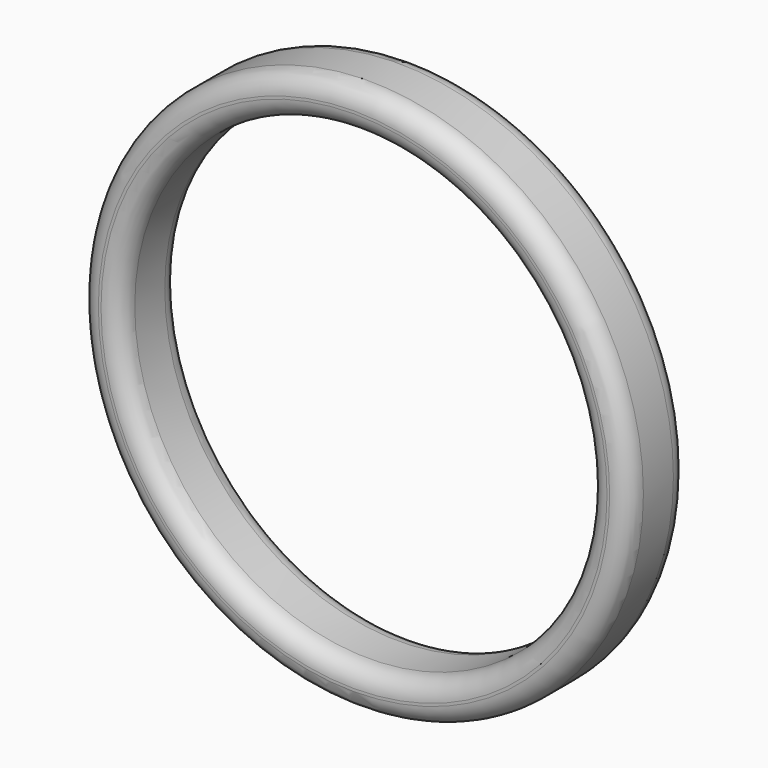
from build123d import *

# Parameters (mm, degrees)
F0_R     = 26.035
F0_R_2   = 22.225
F1_DEPTH = 7.112
F2_R     = 1.778


with BuildPart() as f1:
    # F0 (on Front) → F1 (new body)
    with BuildSketch(Plane.XZ):
        Circle(F0_R)
        Circle(F0_R_2, mode=Mode.SUBTRACT)
    extrude(amount=F1_DEPTH)

    # F2
    f2_edges = [f1.edges().sort_by_distance(p)[0] for p in [
        (-26.035, -7.112, 0),
        (-22.225, -7.112, 0),
        (-26.035, 0, 0),
        (-22.225, 0, 0),
    ]]
    fillet(f2_edges, radius=F2_R)


solid = f1.part
